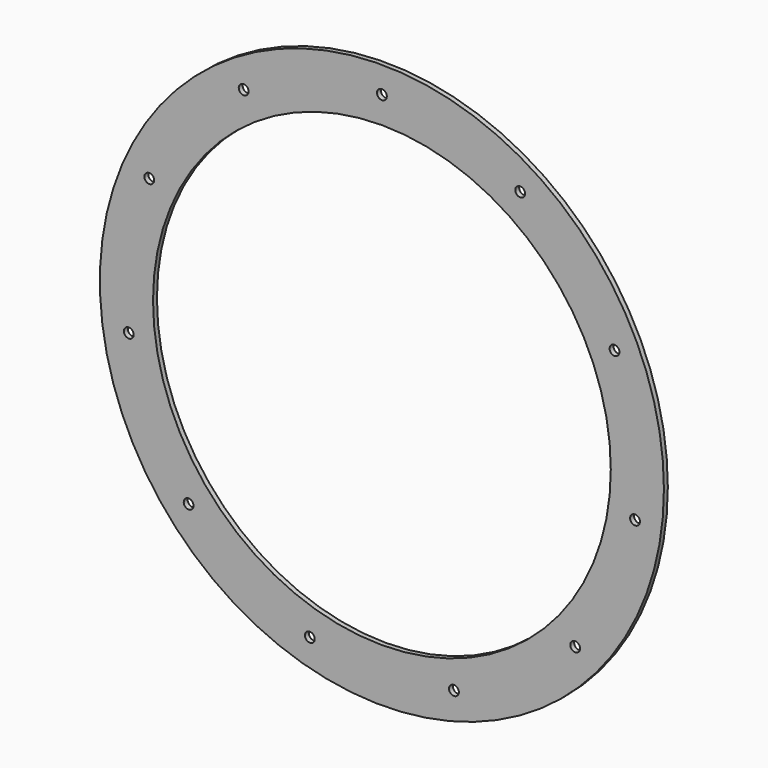
from build123d import *

# Parameters (mm, degrees)
F0_R            = 172.5
F0_R_2          = 140
F1_DEPTH        = 3
F2_R            = 3
F3_DEPTH        = 25
F3_COPIES_COUNT = 11


# Not quite as in the source:
# - a pattern or mirror of a feature is missing from the dataset's text; its kind, count and spacing are read off the source's solid


with BuildPart() as f1:
    # F0 (on Front) → F1 (new body)
    with BuildSketch(Plane.XZ):
        Circle(F0_R)
        Circle(F0_R_2, mode=Mode.SUBTRACT)
    extrude(amount=F1_DEPTH)

    # F2 (on face) → F3 (cut)
    with BuildSketch(Plane.XZ.offset(3)):
        with Locations((0, 156.4114242792)):
            Circle(F2_R)
    f3 = extrude(amount=-F3_DEPTH, mode=Mode.SUBTRACT)

    # F3_copies: F3 ×11 about axis
    f3_copies_axis = Axis((0, 0, 0), (0, 1, 0))
    for i in range(1, F3_COPIES_COUNT):
        add(f3.rotate(f3_copies_axis, i * 360 / F3_COPIES_COUNT), mode=Mode.SUBTRACT)


solid = f1.part
